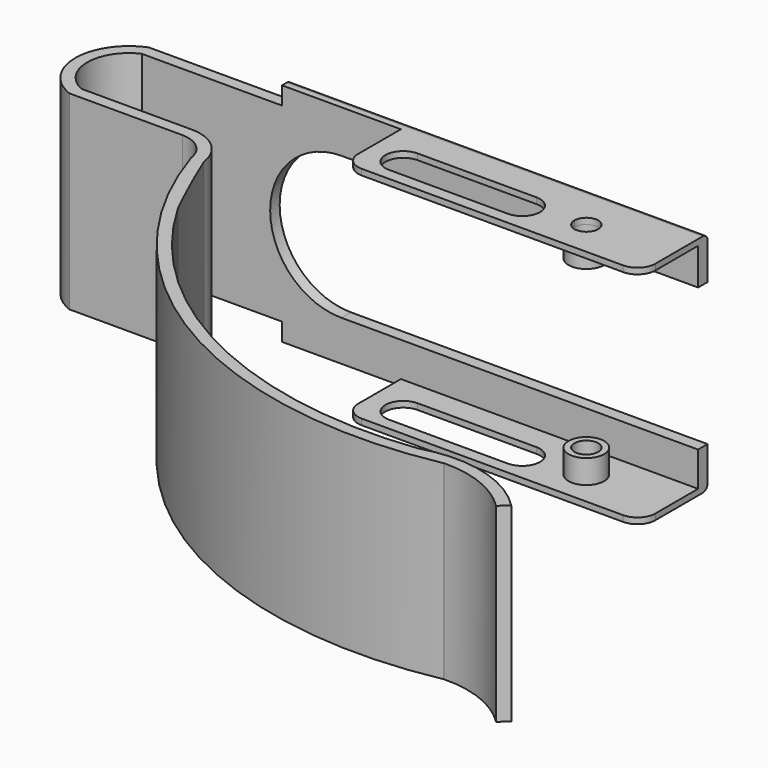
from build123d import *

# Parameters (mm, degrees)
F1_DEPTH  = 16
F2_W      = 70
F2_H      = 3
F3_DEPTH  = 2
F4_W      = 50
F4_H      = 2
F4_H_2    = 12
F5_DEPTH  = 1
F6_R      = 1
F9_DEPTH  = 2
F11_DEPTH = 38.001
F13_D     = 4
F13_DEPTH = 50
F13_TIP   = 1.2017212381
F14_R     = 3
F14_R_2   = 2
F15_DEPTH = 5
F16_R     = 3


# Not quite as in the source:
# - a pattern or mirror of a feature is missing from the dataset's text; its kind, count and spacing are read off the source's solid


with BuildPart() as f1:
    # F0 (on Top) → F1 (new body)
    with BuildSketch(Plane.XY):
        with BuildLine():
            Line((94, 38.2990682213), (94, 40.2990682213))
            Line((94, 40.2990682213), (0, 40.2990682213))
            ThreePointArc((0, 40.2990682213), (-5.6829599791, 31.9326325705), (0, 23.5661969196))
            Line((0, 23.5661969196), (19, 23.5661969196))
            ThreePointArc((19, 23.5661969196), (22.2913263859, 22.330127129), (23.9553291252, 19.2330651681))
            ThreePointArc((23.9553291252, 19.2330651681), (55.0865893222, -19.5660123964), (104.1299821488, -27.8888365183))
            Line((104.1299821488, -27.8888365183), (104.1769053316, -27.8687567031))
            ThreePointArc((104.1769053316, -27.8687567031), (111.1768871923, -29.1372905243), (117.1067956471, -33.0673172193))
            Line((117.1067956471, -33.0673172193), (118.5684373125, -31.7009317787))
            ThreePointArc((118.5684373125, -31.7009317787), (109.440201014, -26.4706046683), (98.9222178887, -26.7009317787))
            ThreePointArc((98.9222178887, -26.7009317787), (60.1395132052, -20.0357341509), (31.5428701215, 6.9967471693))
            ThreePointArc((31.5428701215, 6.9967471693), (28.6246292953, 13.1964823258), (25.9374607753, 19.4998124675))
            ThreePointArc((25.9374607753, 19.4998124675), (23.6078569403, 23.8356992128), (19, 25.5661969196))
            Line((19, 25.5661969196), (0.4069717908, 25.5661969196))
            ThreePointArc((0.4069717908, 25.5661969196), (-3.6829599791, 31.9326325705), (0.4069717908, 38.2990682213))
            Line((0.4069717908, 38.2990682213), (94, 38.2990682213))
        make_face()
    extrude(amount=F1_DEPTH)

    # F2 (on face) → F3 (join)
    with BuildSketch(Plane(origin=(0, 40.2990682213, 0), x_dir=(-1, 0, 0), z_dir=(0, 1, 0))):
        with Locations((-59, 17.5)):
            Rectangle(F2_W, F2_H)
    extrude(amount=-F3_DEPTH)

    # F4 (on face) → F5 (join)
    with BuildSketch(Plane.XY.offset(19)):
        with Locations((69, 39.2990682213)):
            Rectangle(F4_W, F4_H)
        with Locations((69, 32.2990682213)):
            Rectangle(F4_W, F4_H_2)
    extrude(amount=-F5_DEPTH)

    # F6
    f6_edges = [f1.edges().sort_by_distance(p)[0] for p in [
        (59, 40.299068, 19),
    ]]
    fillet(f6_edges, radius=F6_R)

    # F7: F1 across face


with BuildPart() as f1_1:
    add(f1.part)
    add(f1.part.mirror(Plane(origin=(48.2414959272, 12.2129217621, 0), x_dir=(1, 0, 0), z_dir=(0, 0, -1))))

    # F8 (on face) → F9 (cut)
    with BuildSketch(Plane(origin=(0, 40.2990682213, 0), x_dir=(-1, 0, 0), z_dir=(0, 1, 0))):
        with BuildLine():
            Line((-34, 11.8147813603), (-94, 11.8147813603))
            Line((-94, 11.8147813603), (-94, -12.1852186397))
            Line((-94, -12.1852186397), (-34, -12.1852186397))
            ThreePointArc((-34, -12.1852186397), (-22, -0.1852186397), (-34, 11.8147813603))
        make_face()
    extrude(amount=-F9_DEPTH, mode=Mode.SUBTRACT)

    # F10 (on face) → F11 (cut, through all)
    with BuildSketch(Plane.XY.offset(19)):
        with BuildLine():
            ThreePointArc((50, 34.2990682213), (47, 31.2990682213), (50, 28.2990682213))
            Line((50, 28.2990682213), (70, 28.2990682213))
            ThreePointArc((70, 28.2990682213), (73, 31.2990682213), (70, 34.2990682213))
            Line((70, 34.2990682213), (50, 34.2990682213))
        make_face()
    extrude(amount=-F11_DEPTH, mode=Mode.SUBTRACT)

    # F13
    with Locations(Plane.XY.offset(19)):
        with Locations((80, 32.2990682213)):
            Hole(F13_D / 2, depth=F13_DEPTH)
            with Locations((0, 0, -(F13_DEPTH + F13_TIP / 2))):  # 118° drill point
                Cone(0, F13_D / 2, F13_TIP, mode=Mode.SUBTRACT)

    # F14 (on face) → F15 (join)
    with BuildSketch(Plane.XY.offset(19)):
        with Locations((80, 32.2990682213)):
            Circle(F14_R)
        with Locations((80, 32.2990682213)):
            Circle(F14_R_2, mode=Mode.SUBTRACT)
    f15 = extrude(amount=-F15_DEPTH)

    # F15_copies: F15 across plane
    add(f15.mirror(Plane(origin=(0, 0, 0), x_dir=(-1, 0, 0), z_dir=(0, 0, -1))))

    # F16
    f16_edges = [f1_1.edges().sort_by_distance(p)[0] for p in [
        (44, 26.299068, 18.5),
        (44, 26.299068, -18.5),
        (94, 26.299068, -18.5),
        (94, 26.299068, 18.5),
    ]]
    fillet(f16_edges, radius=F16_R)


solid = f1_1.part
